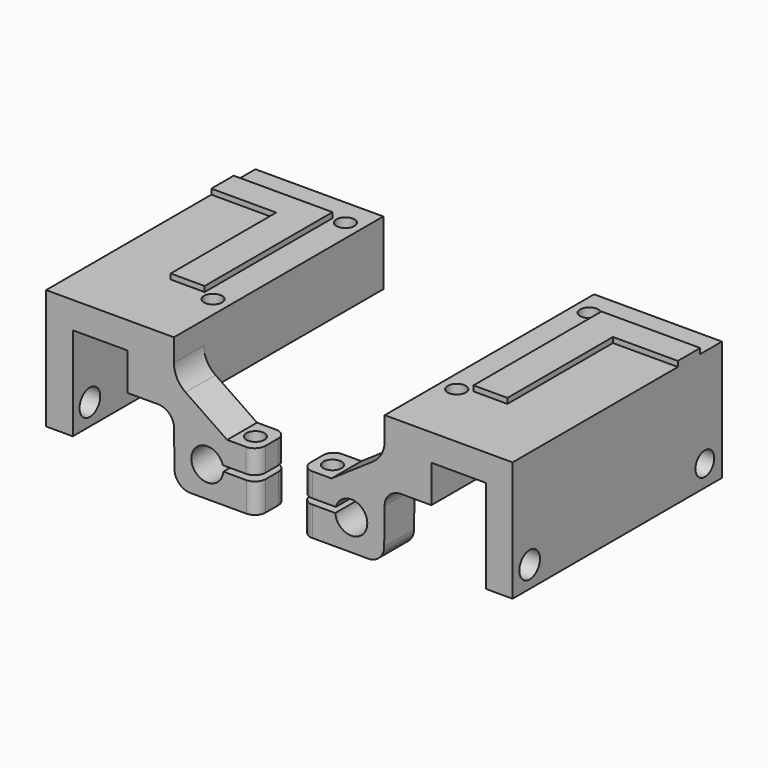
from build123d import *

# Parameters (mm, degrees)
F1_DEPTH      = 7
F2_DEPTH      = 42
F3_R          = 1.7
F3_R_2        = 11
F4_DEPTH      = 12.001
F5_R          = 3
F6_DEPTH      = 10
F7_DEPTH      = 12.001
F8_R          = 1.4
F9_DEPTH      = 10.9920075553
F8_R_2        = 1.7
F10_DEPTH     = 4.4348209087
F11_R         = 5
F12_R         = 3
F13_R         = 3
F14_R         = 2
F15_R         = 2.2
F15_R_2       = 2.4255023423
F16_DEPTH     = 6
F17_TEXT_SIZE = 41.9437823343
F18_DEPTH     = 1


# Not quite as in the source:
# - a feature names something its author has since deleted; it is built from what else it names
# - Text() gives the source's letters only with a copy of the font that has no kerning and outlines rounded to 1/6400 em; it was checked with that copy


with BuildPart() as f1:
    # F0 (on Front) → F1 (new body)
    with BuildSketch(Plane.XZ):
        Polygon((-18.6721007523, 29.8099789735), (-18.6721007523, 7.3259699669), (-13.6721007523, 7.3259699669), (-13.6721007523, 24.8099789735), (-3.4721007523, 24.8099789735), (-3.4721007523, 17.8099789735), (5.2637966118, 17.8099789735), (5.2637966118, 22.9406704692), (5.2637966118, 29.8099789735), align=None)
        Polygon((15.2301751077, 16.1394868046), (5.2637966118, 22.9406704692), (5.2637966118, 17.8099789735), (5.3940201178, 5.1484792493), (20.8186601057, 5.1484792493), (20.8186601057, 10.6682249423), (13.4860510706, 10.6682249423), (13.4860510706, 11.7046658959), (20.7896428882, 11.7046658959), (20.7896428882, 16.1394868046), align=None)
    extrude(amount=F1_DEPTH)

    # F0 (on Front) → F2 (join)
    with BuildSketch(Plane.XZ):
        Polygon((-18.6721007523, 29.8099789735), (-18.6721007523, 7.3259699669), (-13.6721007523, 7.3259699669), (-13.6721007523, 24.8099789735), (-3.4721007523, 24.8099789735), (-3.4721007523, 17.8099789735), (5.2637966118, 17.8099789735), (5.2637966118, 22.9406704692), (5.2637966118, 29.8099789735), align=None)
    extrude(amount=-F2_DEPTH)

    # F3 (on face) → F4 (cut, through all)
    with BuildSketch(Plane(origin=(0, 0, 17.8099789735), x_dir=(1, 0, 0), z_dir=(0, 0, -1))):
        with Locations((2.1850741468, -6)):
            Circle(F3_R)
        with Locations((2.1850741468, -37)):
            Circle(F3_R)
        with Locations((17.6850741468, -21.5)):
            Circle(F3_R_2)
    extrude(amount=-F4_DEPTH, mode=Mode.SUBTRACT)

    # F5 (on face) → F6 (cut)
    with BuildSketch(Plane.XZ.offset(7)):
        with Locations((11.5278992477, 10.8989789735)):
            Circle(F5_R)
    extrude(amount=-F6_DEPTH, mode=Mode.SUBTRACT)

    # F3 (on face) → F7 (cut, through all)
    with BuildSketch(Plane(origin=(0, 0, 17.8099789735), x_dir=(1, 0, 0), z_dir=(0, 0, -1))):
        with Locations((2.1850741468, -6)):
            Circle(F3_R)
        with Locations((2.1850741468, -37)):
            Circle(F3_R)
        with Locations((17.6850741468, -21.5)):
            Circle(F3_R_2)
    extrude(amount=-F7_DEPTH, mode=Mode.SUBTRACT)

    # F8 (on face) → F9 (cut, through all)
    with BuildSketch(Plane.XY.offset(16.1394868046)):
        with Locations((17.7896428882, -3.5767070949)):
            Circle(F8_R)
    extrude(amount=-F9_DEPTH, mode=Mode.SUBTRACT)

    # F8 (on face) → F10 (cut, through all)
    with BuildSketch(Plane.XY.offset(16.1394868046)):
        with Locations((17.7896428882, -3.5767070949)):
            Circle(F8_R_2)
        with Locations((17.7896428882, -3.5767070949)):
            Circle(F8_R, mode=Mode.SUBTRACT)
    extrude(amount=-F10_DEPTH, mode=Mode.SUBTRACT)

    # F11
    f11_edges = [f1.edges().sort_by_distance(p)[0] for p in [
        (5.263797, -3.5, 22.94067),
    ]]
    fillet(f11_edges, radius=F11_R)

    # F12
    f12_edges = [f1.edges().sort_by_distance(p)[0] for p in [
        (5.263797, -3.5, 17.809979),
    ]]
    fillet(f12_edges, radius=F12_R)

    # F13
    f13_edges = [f1.edges().sort_by_distance(p)[0] for p in [
        (5.39402, -3.5, 5.148479),
    ]]
    fillet(f13_edges, radius=F13_R)

    # F14
    f14_edges = [f1.edges().sort_by_distance(p)[0] for p in [
        (20.789643, -7, 13.922076),
        (20.81866, -7, 7.908352),
        (20.789643, 0, 13.922076),
        (20.81866, 0, 7.908352),
    ]]
    fillet(f14_edges, radius=F14_R)

    # F15 (on face) → F16 (cut)
    with BuildSketch(Plane(origin=(-18.6721007523, 0, 0), x_dir=(0, -1, 0), z_dir=(-1, 0, 0))):
        with Locations((-38, 11.3259699669)):
            Circle(F15_R)
        with Locations((3, 11.3259699669)):
            Circle(F15_R_2)
    extrude(amount=-F16_DEPTH, mode=Mode.SUBTRACT)

    # F17 (on face) → F18 (join)
    with BuildSketch(Plane.XY.offset(29.8099789735)):
        with Locations(Location((3.5908724648, 36.9253193088), (0, 0, 180))):
            Text('L', F17_TEXT_SIZE, font='Open Sans', font_style=FontStyle.BOLD, text_align=(TextAlign.LEFT, TextAlign.BOTTOM))
    extrude(amount=F18_DEPTH)


with BuildPart() as f19_1:
    # F19: instance of F1
    add(f1.part.mirror(Plane.YZ))


with BuildPart() as f19_1_1:
    # F20: moved
    add(f19_1.part.moved(Location((50, 0, 0))))


solid = Compound([f1.part, f19_1_1.part])
